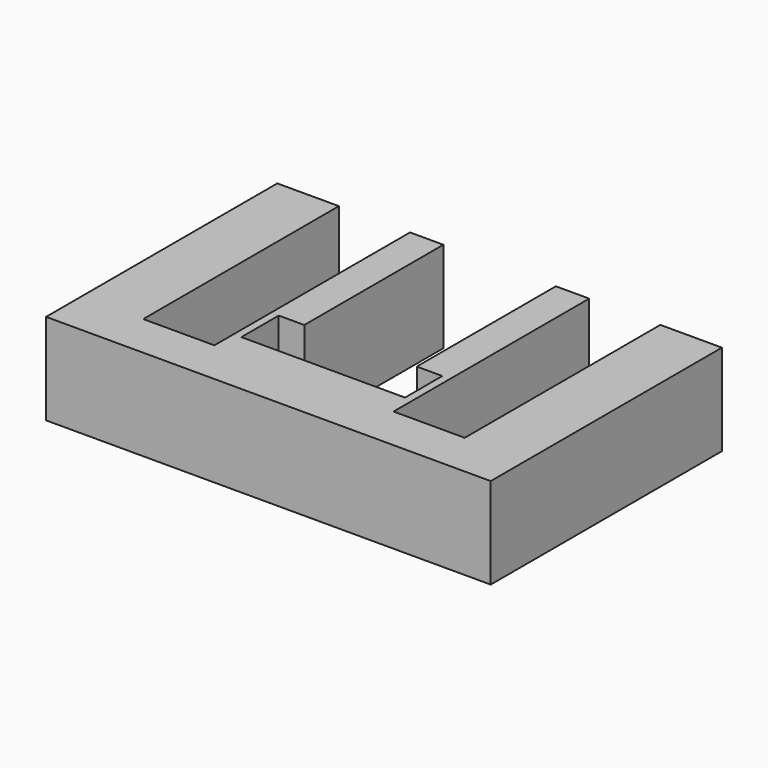
from build123d import *

# Parameters (mm, degrees)
F1_DEPTH = 5.1
F2_W     = 3.2
F2_H     = 3.2
F4_DEPTH = 11
F3_W     = 3.2
F3_H     = 3.2
F5_DEPTH = 11
F6_DEPTH = 1


# Not quite as in the source:
# - a feature names something its author has since deleted; it is built from what else it names


with BuildPart() as f1:
    # F0 (on Top) → F1 (new body)
    with BuildSketch(Plane.XY):
        Polygon((-17.8524617243, -0.2032842353), (-25.3224617243, -0.2032842353), (-25.3224617243, -13.2032842353), (-5.3224617243, -13.2032842353), (-5.3224617243, -0.2032842353), (-12.7924617243, -0.2032842353), (-12.7924617243, -8.0232842353), (-11.6424617243, -8.0232842353), (-11.6424617243, -10.1232842353), (-19.0024617243, -10.1232842353), (-19.0024617243, -8.0232842353), (-17.8524617243, -8.0232842353), align=None)
    extrude(amount=F1_DEPTH)

    # F2 (on face) → F4 (cut)
    with BuildSketch(Plane(origin=(0, -0.2032842353, 0), x_dir=(-1, 0, 0), z_dir=(0, 1, 0))):
        with Locations((9.6924617243, 2.55)):
            Rectangle(F2_W, F2_H)
    extrude(amount=-F4_DEPTH, mode=Mode.SUBTRACT)

    # F3 (on face) → F5 (cut)
    with BuildSketch(Plane(origin=(0, -0.2032842353, 0), x_dir=(-1, 0, 0), z_dir=(0, 1, 0))):
        with Locations((20.9524617243, 2.55)):
            Rectangle(F3_W, F3_H)
    extrude(amount=-F5_DEPTH, mode=Mode.SUBTRACT)

    # F6 (cut): a face of the model
    f6_faces = [f1.faces().sort_by_distance(p)[0] for p in [
        (-19.2409989331, -9.0732842353, 5.1),
    ]]
    extrude(f6_faces, amount=-F6_DEPTH, mode=Mode.SUBTRACT)


solid = f1.part
